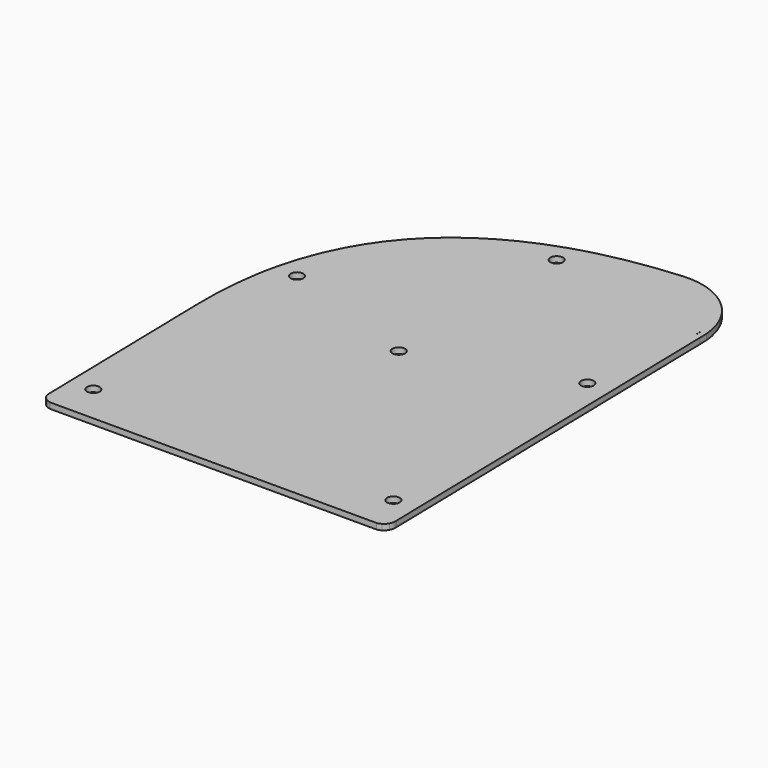
from build123d import *

# Parameters (mm, degrees)
F0_R     = 1.65
F1_DEPTH = 1.5


# Not quite as in the source:
# - the dataset's text gives a spline's control points without its knots; the knots are read off the source's solid
# - a feature names something its author has since deleted; it is built from what else it names


with BuildPart() as f1:
    # F0 (on Top) → F1 (new body)
    with BuildSketch(Plane.XY):
        with BuildLine():
            add(Edge.make_bspline(
                [(-1.4834199291, 56.9861769818), (-24.0434344456, 49.5840490447), (-39.5518296707, 34.0581899342), (-43.7697110627, 8.0514126658)],
                knots=[23.6646194308, 23.6646194308, 23.6646194308, 23.6646194308, 87.6009906021, 87.6009906021, 87.6009906021, 87.6009906021], degree=3))
            Line((-43.7697110627, 8.0514126658), (-43.3999866886, -9.4545040952))
            add(Edge.make_bspline(
                [(-41.6084588868, 11.4552943961), (-41.9131684463, 10.0195533179), (-43.0811996644, 3.5961523714), (-43.5251604122, -3.527708515), (-43.3999866886, -9.4545040952)],
                knots=[0.8378421155, 0.8378421155, 0.8378421155, 0.8378421155, 0.875, 1, 1, 1, 1], degree=3))
            ThreePointArc((-41.6084588868, 11.4552943961), (-41.6746745213, 14.1216598486), (-40.360654899, 16.442703077))
            add(Edge.make_bspline(
                [(-3.9361636907, 54.5413772398), (-7.7396177388, 53.1307994352), (-15.2958477205, 49.6198124705), (-25.1166954602, 42.4854415502), (-33.2620494576, 33.0539884408), (-37.9347962076, 23.9582519777), (-39.9020549062, 18.0232145314), (-40.360654899, 16.442703077)],
                knots=[0.2629122118, 0.2629122118, 0.2629122118, 0.2629122118, 0.375, 0.5, 0.625, 0.75, 0.7934924029, 0.7934924029, 0.7934924029, 0.7934924029], degree=3))
            ThreePointArc((-3.9361636907, 54.5413772398), (-1.5789362683, 56.2022473749), (1.3034460345, 56.2852111481))
            add(Edge.make_bspline(
                [(3.7948607758, 56.9861769817), (2.9552380235, 56.7627416597), (2.1246988708, 56.5291170771), (1.3034460345, 56.2852111481)],
                knots=[0.1898045831, 0.1898045831, 0.1898045831, 0.1898045831, 0.2127848006, 0.2127848006, 0.2127848006, 0.2127848006], degree=3))
            Line((3.7948607758, 56.9861769818), (-1.4834199291, 56.9861769818))
        make_face()
        with BuildLine():
            add(Edge.make_bspline(
                [(-40.360654899, 16.442703077), (-40.8282946823, 14.8310370372), (-41.2447734518, 13.1689200516), (-41.6084588868, 11.4552943961)],
                knots=[0.7934924029, 0.7934924029, 0.7934924029, 0.7934924029, 0.8378421155, 0.8378421155, 0.8378421155, 0.8378421155], degree=3))
            ThreePointArc((-41.6084588868, 11.4552943961), (-36.6028372853, 7.9130121651), (-31.9301505005, 11.884159258))
            ThreePointArc((-31.9301505005, 11.884159258), (-31.8507431164, 12.393400412), (-31.8241799079, 12.9081105068))
            ThreePointArc((-31.8241799079, 12.9081105068), (-34.9113776383, 17.5277628181), (-40.360654899, 16.442703077))
        make_face()
        with Locations((-36.8241799079, 12.9081105068)):
            Circle(F0_R, mode=Mode.SUBTRACT)
        with BuildLine():
            ThreePointArc((-40.360654899, 16.442703077), (-41.6746745213, 14.1216598486), (-41.6084588868, 11.4552943961))
            add(Edge.make_bspline(
                [(-40.360654899, 16.442703077), (-40.8282946823, 14.8310370372), (-41.2447734518, 13.1689200516), (-41.6084588868, 11.4552943961)],
                knots=[0.7934924029, 0.7934924029, 0.7934924029, 0.7934924029, 0.8378421155, 0.8378421155, 0.8378421155, 0.8378421155], degree=3))
        make_face()
        with BuildLine():
            ThreePointArc((-4.0125837516, 2.9831479408), (-4.2957315609, 2.5586501044), (-4.534139997, 2.1075043268))
            ThreePointArc((-4.534139997, 2.1075043268), (-1.0791895142, -4.8821460438), (5, 0))
            ThreePointArc((5, 0), (4.9178269212, 0.9027615264), (4.6740086506, 1.7758499751))
            ThreePointArc((4.6740086506, 1.7758499751), (4.4710674532, 2.2382037059), (4.2225292185, 2.6777316891))
            ThreePointArc((4.2225292185, 2.6777316891), (0.1853079774, 4.9965649154), (-4.0125837516, 2.9831479408))
        make_face()
        Circle(F0_R, mode=Mode.SUBTRACT)
        with BuildLine():
            ThreePointArc((33.856602495, 11.8901119011), (38.3087519579, 7.9829804344), (43.3659270117, 11.0671807542))
            Line((43.3659270117, 11.0671807542), (43.281700799, 15.0551706498))
            ThreePointArc((43.281700799, 15.0551706498), (37.6421734995, 17.842387831), (33.7401541423, 12.9081105068))
            ThreePointArc((33.7401541423, 12.9081105068), (33.7722325318, 12.3961204004), (33.856602495, 11.8901119011))
        make_face()
        with Locations((38.8260431298, 12.9081105068)):
            Circle(F0_R, mode=Mode.SUBTRACT)
        with BuildLine():
            Line((43.281700799, 15.0551706498), (43.3659270117, 11.0671807542))
            ThreePointArc((43.3659270117, 11.0671807542), (43.6454694966, 11.9975237522), (43.7398377061, 12.9643622786))
            ThreePointArc((43.7398377061, 12.9643622786), (43.623960732, 14.0345689258), (43.281700799, 15.0551706498))
        make_face()
        with BuildLine():
            Line((43.3659270117, 11.0671807542), (44.6495853815, -49.7121947628))
            ThreePointArc((44.6495853815, -49.7121947628), (45.057929388, -50.8167509251), (45.1966083023, -51.9861769818))
            ThreePointArc((45.1966083023, -51.9861769818), (45.0815382797, -53.0526942652), (44.7416246559, -54.0701218815))
            Line((44.7416246559, -54.0701218815), (44.7906830466, -56.3929660398))
            ThreePointArc((44.7906830466, -56.3929660398), (45.8531698465, -57.3651583436), (46.3401743003, -58.7204674365))
            Line((46.3401743003, -58.7204674365), (44.1920061045, 42.9922035609))
            ThreePointArc((44.1920061045, 42.9922035609), (43.7876646895, 39.7863466035), (42.8245210763, 36.7019722436))
            Line((42.8245210763, 36.7019722436), (43.281700799, 15.0551706498))
            ThreePointArc((43.281700799, 15.0551706498), (43.623960732, 14.0345689258), (43.7398377061, 12.9643622786))
            ThreePointArc((43.7398377061, 12.9643622786), (43.6454694966, 11.9975237522), (43.3659270117, 11.0671807542))
        make_face()
        with BuildLine():
            ThreePointArc((42.8245210763, 36.7019722436), (43.7876646895, 39.7863466035), (44.1920061045, 42.9922035609))
            Line((44.1920061045, 42.9922035609), (44.1473284715, 45.1076251571))
            ThreePointArc((44.1473284715, 45.1076251571), (43.6079928038, 48.2935516862), (42.5154823554, 51.3345107013))
            Line((42.5154823554, 51.3345107013), (42.6486009917, 45.0315349493))
            ThreePointArc((42.6486009917, 45.0315349493), (42.6904501625, 44.3488552909), (42.704407636, 43.6650365591))
            ThreePointArc((42.704407636, 43.6650365591), (42.7011560215, 43.3349282258), (42.6914024401, 43.0049479956))
            Line((42.6914024401, 43.0049479956), (42.8245210763, 36.7019722436))
        make_face()
        with BuildLine():
            ThreePointArc((42.5154823554, 51.3345107013), (40.7462901657, 54.3570465919), (38.43254048, 56.9861769818))
            Line((38.43254048, 56.9861769818), (36.1139913688, 56.9861769818))
            ThreePointArc((36.1139913688, 56.9861769818), (40.6509720914, 51.7028823031), (42.6486009917, 45.0315349493))
            Line((42.6486009917, 45.0315349493), (42.5154823554, 51.3345107013))
        make_face()
        with BuildLine():
            add(Edge.make_bspline(
                [(24.7414019258, 61.8833889583), (24.6406996854, 61.8759974959), (24.5400748401, 61.8685045119), (24.4395276097, 61.8609098839)],
                knots=[1.1865276968, 1.1865276968, 1.1865276968, 1.1865276968, 1.425041868, 1.425041868, 1.425041868, 1.425041868], degree=3))
            ThreePointArc((24.4395276097, 61.8609098839), (20.5940502811, 61.1210933261), (16.9947819167, 59.5782739378))
            add(Edge.make_bspline(
                [(24.5558527888, 60.365406788), (21.9807579148, 60.170918351), (19.4591236125, 59.9091209792), (16.9947819167, 59.5782739378)],
                knots=[0.0141040109, 0.0141040109, 0.0141040109, 0.0141040109, 0.0753203459, 0.0753203459, 0.0753203459, 0.0753203459], degree=3))
            ThreePointArc((24.5558527888, 60.365406788), (24.7014970491, 60.3768935027), (24.8472359143, 60.3871100752))
            ThreePointArc((24.8472359143, 60.3871100752), (30.7889811323, 59.7082164359), (36.1139913688, 56.9861769818))
            Line((36.1139913688, 56.9861769818), (38.43254048, 56.9861769818))
            ThreePointArc((38.43254048, 56.9861769818), (32.0955113167, 60.8565088809), (24.7414019258, 61.8833889583))
        make_face()
        with BuildLine():
            add(Edge.make_bspline(
                [(24.4395276097, 61.8609098839), (15.0642862312, 61.1527703288), (6.3638379536, 59.5609273996), (-1.4834199291, 56.9861769818)],
                knots=[1.425041868, 1.425041868, 1.425041868, 1.425041868, 23.6646194308, 23.6646194308, 23.6646194308, 23.6646194308], degree=3))
            Line((-1.4834199291, 56.9861769818), (3.7948607758, 56.9861769818))
            add(Edge.make_bspline(
                [(16.9947819167, 59.5782739378), (12.3860728261, 58.9595375953), (7.9777441733, 58.0993005798), (3.7948607758, 56.9861769817)],
                knots=[0.0753203459, 0.0753203459, 0.0753203459, 0.0753203459, 0.1898045831, 0.1898045831, 0.1898045831, 0.1898045831], degree=3))
            ThreePointArc((16.9947819167, 59.5782739378), (20.5940502811, 61.1210933261), (24.4395276097, 61.8609098839))
        make_face()
        with BuildLine():
            ThreePointArc((5, 51.4580972655), (3.969712217, 54.4980618893), (1.3034460345, 56.2852111481))
            add(Edge.make_bspline(
                [(1.3034460345, 56.2852111481), (-0.0265278019, 55.8902188998), (-1.7851459927, 55.3218605731), (-3.4980160121, 54.7038720098), (-3.9361636907, 54.5413772398)],
                knots=[0.2127848006, 0.2127848006, 0.2127848006, 0.2127848006, 0.25, 0.2629122118, 0.2629122118, 0.2629122118, 0.2629122118], degree=3))
            ThreePointArc((-3.9361636907, 54.5413772398), (-1.6308251817, 46.731533056), (5, 51.4580972655))
        make_face()
        with Locations((0, 51.4580972655)):
            Circle(F0_R, mode=Mode.SUBTRACT)
        with BuildLine():
            add(Edge.make_bspline(
                [(1.3034460345, 56.2852111481), (-0.0265278019, 55.8902188998), (-1.7851459927, 55.3218605731), (-3.4980160121, 54.7038720098), (-3.9361636907, 54.5413772398)],
                knots=[0.2127848006, 0.2127848006, 0.2127848006, 0.2127848006, 0.25, 0.2629122118, 0.2629122118, 0.2629122118, 0.2629122118], degree=3))
            ThreePointArc((1.3034460345, 56.2852111481), (-1.5789362683, 56.2022473749), (-3.9361636907, 54.5413772398))
        make_face()
        with BuildLine():
            Line((-44.8996522607, -9.4861769818), (-43.857959234, -58.8088418975))
            ThreePointArc((-43.857959234, -58.8088418975), (-43.423907092, -57.4454091965), (-42.4076946201, -56.4381047717))
            Line((-42.4076946201, -56.4381047717), (-42.4536350786, -54.2628902097))
            ThreePointArc((-42.4536350786, -54.2628902097), (-43.0009389284, -52.0917532702), (-42.5457909037, -49.8994445807))
            Line((-42.5457909037, -49.8994445807), (-43.3999866886, -9.4545040952))
            Line((-43.3999866886, -9.4545040952), (-43.7697110627, 8.0514126658))
            add(Edge.make_bspline(
                [(-43.7697110627, 8.0514126658), (-44.6436982543, 2.6625484195), (-45.0329161364, -3.1763243502), (-44.8996522607, -9.4861769818)],
                knots=[87.6009906021, 87.6009906021, 87.6009906021, 87.6009906021, 100.8492458966, 100.8492458966, 100.8492458966, 100.8492458966], degree=3))
        make_face()
        with BuildLine():
            ThreePointArc((-42.4536350786, -54.2628902097), (-41.8118478695, -55.2243042636), (-40.9664335917, -56.0126458797))
            ThreePointArc((-40.9664335917, -56.0126458797), (-39.732615879, -56.2327544404), (-38.6963915431, -56.9377317823))
            ThreePointArc((-38.6963915431, -56.9377317823), (-34.7211764635, -55.75921881), (-33.0020536879, -51.9861769818))
            ThreePointArc((-33.0020536879, -51.9861769818), (-36.9340382571, -47.1015743327), (-42.5457909037, -49.8994445807))
            Line((-42.5457909037, -49.8994445807), (-42.4536350786, -54.2628902097))
        make_face()
        with Locations((-38.0020536879, -51.9861769818)):
            Circle(F0_R, mode=Mode.SUBTRACT)
        with BuildLine():
            Line((-43.857959234, -58.8088418975), (-43.8467581028, -59.339199334))
            ThreePointArc((-43.8467581028, -59.339199334), (-43.7200551284, -59.9314469487), (-43.4769800964, -60.4861769818))
            Line((-43.4769800964, -60.4861769818), (-42.3221994709, -60.4861769818))
            Line((-42.3221994709, -60.4861769818), (-42.4076946201, -56.4381047717))
            ThreePointArc((-42.4076946201, -56.4381047717), (-43.423907092, -57.4454091965), (-43.857959234, -58.8088418975))
        make_face()
        with BuildLine():
            ThreePointArc((-43.4769800964, -60.4861769818), (-42.96891188, -61.1492867627), (-42.2976915724, -61.6465906868))
            Line((-42.2976915724, -61.6465906868), (-42.3221994709, -60.4861769818))
            Line((-42.3221994709, -60.4861769818), (-43.4769800964, -60.4861769818))
        make_face()
        with BuildLine():
            ThreePointArc((-42.2976915724, -61.6465906868), (-41.7892239121, -61.8649359932), (-41.2493029391, -61.9861769818))
            Line((-41.2493029391, -61.9861769818), (-40.4802432502, -61.9861769818))
            ThreePointArc((-40.4802432502, -61.9861769818), (-39.1891812794, -61.49937465), (-38.2525660929, -60.4861769818))
            Line((-38.2525660929, -60.4861769818), (-42.3221994709, -60.4861769818))
            Line((-42.3221994709, -60.4861769818), (-42.2976915724, -61.6465906868))
        make_face()
        with BuildLine():
            ThreePointArc((-38.2525660929, -60.4861769818), (-39.1891812794, -61.49937465), (-40.4802432502, -61.9861769818))
            Line((-40.4802432502, -61.9861769818), (42.8588795725, -61.9861769818))
            ThreePointArc((42.8588795725, -61.9861769818), (41.6256295111, -61.4783601673), (40.7343629083, -60.4861769818))
            Line((40.7343629083, -60.4861769818), (-38.2525660929, -60.4861769818))
        make_face()
        with BuildLine():
            ThreePointArc((40.7343629083, -60.4861769818), (41.6256295111, -61.4783601673), (42.8588795725, -61.9861769818))
            Line((42.8588795725, -61.9861769818), (43.8530039724, -61.9861769818))
            ThreePointArc((43.8530039724, -61.9861769818), (44.3949796267, -61.8419625935), (44.9006425936, -61.5993922664))
            Line((44.9006425936, -61.5993922664), (44.8771315242, -60.4861769818))
            Line((44.8771315242, -60.4861769818), (40.7343629083, -60.4861769818))
        make_face()
        with BuildLine():
            Line((44.7906830466, -56.3929660398), (44.8771315242, -60.4861769818))
            Line((44.8771315242, -60.4861769818), (45.9775206366, -60.4861769818))
            ThreePointArc((45.9775206366, -60.4861769817), (46.2357482904, -59.8683050946), (46.3504824841, -59.2085450967))
            Line((46.3504824841, -59.2085450967), (46.3401743003, -58.7204674365))
            ThreePointArc((46.3401743003, -58.7204674365), (45.8531698465, -57.3651583436), (44.7906830466, -56.3929660398))
        make_face()
        with BuildLine():
            Line((44.8771315242, -60.4861769818), (44.9006425936, -61.5993922664))
            ThreePointArc((44.9006425936, -61.5993922664), (45.5121615367, -61.1134790926), (45.9775206366, -60.4861769817))
            Line((45.9775206366, -60.4861769818), (44.8771315242, -60.4861769818))
        make_face()
        with BuildLine():
            ThreePointArc((44.6495853815, -49.7121947628), (35.6747286545, -49.8524936757), (41.2725763461, -56.8690340111))
            ThreePointArc((41.2725763461, -56.8690340111), (42.1278630999, -56.2905225817), (43.1286349994, -56.0362658014))
            ThreePointArc((43.1286349994, -56.0362658014), (44.062222571, -55.1574584776), (44.7416246559, -54.0701218815))
            Line((44.7416246559, -54.0701218815), (44.6495853815, -49.7121947628))
        make_face()
        with Locations((40.1966083023, -51.9861769818)):
            Circle(F0_R, mode=Mode.SUBTRACT)
        with BuildLine():
            ThreePointArc((41.2725763461, -56.8690340111), (40.3886103094, -58.5861173938), (40.7343629083, -60.4861769818))
            Line((40.7343629083, -60.4861769818), (44.8771315242, -60.4861769818))
            Line((44.8771315242, -60.4861769818), (44.7906830466, -56.3929660398))
            ThreePointArc((44.7906830466, -56.3929660398), (43.9854521247, -56.0944327255), (43.1286349994, -56.0362658014))
            ThreePointArc((43.1286349994, -56.0362658014), (42.2434060899, -56.5480426984), (41.2725763461, -56.8690340111))
        make_face()
        with BuildLine():
            ThreePointArc((44.7416246559, -54.0701218815), (44.062222571, -55.1574584776), (43.1286349994, -56.0362658014))
            ThreePointArc((43.1286349994, -56.0362658014), (43.9854521247, -56.0944327255), (44.7906830466, -56.3929660398))
            Line((44.7906830466, -56.3929660398), (44.7416246559, -54.0701218815))
        make_face()
        with BuildLine():
            ThreePointArc((43.1286349994, -56.0362658014), (42.1278630999, -56.2905225817), (41.2725763461, -56.8690340111))
            ThreePointArc((41.2725763461, -56.8690340111), (42.2434060899, -56.5480426984), (43.1286349994, -56.0362658014))
        make_face()
        with BuildLine():
            ThreePointArc((45.1966083023, -51.9861769818), (45.057929388, -50.8167509251), (44.6495853815, -49.7121947628))
            Line((44.6495853815, -49.7121947628), (44.7416246559, -54.0701218815))
            ThreePointArc((44.7416246559, -54.0701218815), (45.0815382797, -53.0526942652), (45.1966083023, -51.9861769818))
        make_face()
        with BuildLine():
            ThreePointArc((-42.5457909037, -49.8994445807), (-43.0009389284, -52.0917532702), (-42.4536350786, -54.2628902097))
            Line((-42.4536350786, -54.2628902097), (-42.5457909037, -49.8994445807))
        make_face()
        with BuildLine():
            ThreePointArc((-38.6963915431, -56.9377317823), (-39.732615879, -56.2327544404), (-40.9664335917, -56.0126458797))
            ThreePointArc((-40.9664335917, -56.0126458797), (-39.8889823808, -56.6164577625), (-38.6963915431, -56.9377317823))
        make_face()
        with BuildLine():
            Line((-42.3221994709, -60.4861769818), (-38.2525660929, -60.4861769818))
            ThreePointArc((-38.2525660929, -60.4861769818), (-37.9633406032, -59.7736086221), (-37.8647730947, -59.0109229088))
            ThreePointArc((-37.8647730947, -59.0109229088), (-38.0804289479, -57.8940398922), (-38.6963915431, -56.9377317823))
            ThreePointArc((-38.6963915431, -56.9377317823), (-39.8889823808, -56.6164577625), (-40.9664335917, -56.0126458797))
            ThreePointArc((-40.9664335917, -56.0126458797), (-41.7141353992, -56.1336701087), (-42.4076946201, -56.4381047717))
            Line((-42.4076946201, -56.4381047717), (-42.3221994709, -60.4861769818))
        make_face()
        with BuildLine():
            Line((-42.4536350786, -54.2628902097), (-42.4076946201, -56.4381047717))
            ThreePointArc((-42.4076946201, -56.4381047717), (-41.7141353992, -56.1336701087), (-40.9664335917, -56.0126458797))
            ThreePointArc((-40.9664335917, -56.0126458797), (-41.8118478695, -55.2243042636), (-42.4536350786, -54.2628902097))
        make_face()
        with BuildLine():
            Line((4.6740086506, 1.7758499751), (33.856602495, 11.8901119011))
            ThreePointArc((33.856602495, 11.8901119011), (33.7722325318, 12.3961204004), (33.7401541423, 12.9081105068))
            Line((33.7401541423, 12.9081105068), (4.2225292185, 2.6777316891))
            ThreePointArc((4.2225292185, 2.6777316891), (4.4710674532, 2.2382037059), (4.6740086506, 1.7758499751))
        make_face()
        with BuildLine():
            ThreePointArc((-31.8241799079, 12.9081105068), (-31.8507431164, 12.393400412), (-31.9301505005, 11.884159258))
            Line((-31.9301505005, 11.884159258), (-4.534139997, 2.1075043268))
            ThreePointArc((-4.534139997, 2.1075043268), (-4.2957315609, 2.5586501044), (-4.0125837516, 2.9831479408))
            Line((-4.0125837516, 2.9831479408), (-31.8241799079, 12.9081105068))
        make_face()
        with BuildLine():
            Line((13.4599747919, 56.9861769818), (3.7948607758, 56.9861769818))
            add(Edge.make_bspline(
                [(3.7948607758, 56.9861769817), (2.9552380235, 56.7627416597), (2.1246988708, 56.5291170771), (1.3034460345, 56.2852111481)],
                knots=[0.1898045831, 0.1898045831, 0.1898045831, 0.1898045831, 0.2127848006, 0.2127848006, 0.2127848006, 0.2127848006], degree=3))
            ThreePointArc((1.3034460345, 56.2852111481), (3.969712217, 54.4980618893), (5, 51.4580972655))
            ThreePointArc((5, 51.4580972655), (-1.6308251817, 46.731533056), (-3.9361636907, 54.5413772398))
            add(Edge.make_bspline(
                [(-3.9361636907, 54.5413772398), (-7.7396177388, 53.1307994352), (-15.2958477205, 49.6198124705), (-25.1166954602, 42.4854415502), (-33.2620494576, 33.0539884408), (-37.9347962076, 23.9582519777), (-39.9020549062, 18.0232145314), (-40.360654899, 16.442703077)],
                knots=[0.2629122118, 0.2629122118, 0.2629122118, 0.2629122118, 0.375, 0.5, 0.625, 0.75, 0.7934924029, 0.7934924029, 0.7934924029, 0.7934924029], degree=3))
            ThreePointArc((-40.360654899, 16.442703077), (-34.9113776383, 17.5277628181), (-31.8241799079, 12.9081105068))
            Line((-31.8241799079, 12.9081105068), (-4.0125837516, 2.9831479408))
            ThreePointArc((-4.0125837516, 2.9831479408), (0.1853079774, 4.9965649154), (4.2225292185, 2.6777316891))
            Line((4.2225292185, 2.6777316891), (33.7401541423, 12.9081105068))
            ThreePointArc((33.7401541423, 12.9081105068), (37.6421734995, 17.842387831), (43.281700799, 15.0551706498))
            Line((43.281700799, 15.0551706498), (42.8245210763, 36.7019722436))
            ThreePointArc((42.8245210763, 36.7019722436), (15.5691379077, 28.6425391779), (13.4599747919, 56.9861769817))
        make_face()
        with BuildLine():
            Line((36.1139913688, 56.9861769818), (15.7785239031, 56.9861769818))
            ThreePointArc((15.7785239031, 56.9861769818), (18.2206977798, 28.7938793637), (42.6914024401, 43.0049479956))
            Line((42.6914024401, 43.0049479956), (42.6486009917, 45.0315349493))
            ThreePointArc((42.6486009917, 45.0315349493), (40.6509720914, 51.7028823031), (36.1139913688, 56.9861769818))
        make_face()
        with BuildLine():
            add(Edge.make_bspline(
                [(24.8472359143, 60.3871100752), (24.7500324053, 60.3799711919), (24.6529046285, 60.3727367939), (24.5558527888, 60.365406788)],
                knots=[0.0117968501, 0.0117968501, 0.0117968501, 0.0117968501, 0.0141040109, 0.0141040109, 0.0141040109, 0.0141040109], degree=3))
            ThreePointArc((24.5558527888, 60.365406788), (19.9252576875, 59.3041909814), (15.7785239031, 56.9861769818))
            Line((15.7785239031, 56.9861769818), (36.1139913688, 56.9861769818))
            ThreePointArc((36.1139913688, 56.9861769818), (30.7889811323, 59.7082164359), (24.8472359143, 60.3871100752))
        make_face()
        with BuildLine():
            add(Edge.make_bspline(
                [(16.9947819167, 59.5782739378), (12.3860728261, 58.9595375953), (7.9777441733, 58.0993005798), (3.7948607758, 56.9861769817)],
                knots=[0.0753203459, 0.0753203459, 0.0753203459, 0.0753203459, 0.1898045831, 0.1898045831, 0.1898045831, 0.1898045831], degree=3))
            Line((3.7948607758, 56.9861769818), (13.4599747919, 56.9861769818))
            ThreePointArc((13.4599747919, 56.9861769817), (15.1493083116, 58.3886885079), (16.9947819167, 59.5782739378))
        make_face()
        with BuildLine():
            add(Edge.make_bspline(
                [(24.5558527888, 60.365406788), (21.9807579148, 60.170918351), (19.4591236125, 59.9091209792), (16.9947819167, 59.5782739378)],
                knots=[0.0141040109, 0.0141040109, 0.0141040109, 0.0141040109, 0.0753203459, 0.0753203459, 0.0753203459, 0.0753203459], degree=3))
            ThreePointArc((16.9947819167, 59.5782739378), (15.1493083116, 58.3886885079), (13.4599747919, 56.9861769817))
            Line((13.4599747919, 56.9861769818), (15.7785239031, 56.9861769818))
            ThreePointArc((15.7785239031, 56.9861769818), (19.9252576875, 59.3041909814), (24.5558527888, 60.365406788))
        make_face()
        with BuildLine():
            Line((15.7785239031, 56.9861769818), (13.4599747919, 56.9861769818))
            ThreePointArc((13.4599747919, 56.9861769817), (15.5691379077, 28.6425391779), (42.8245210763, 36.7019722436))
            Line((42.8245210763, 36.7019722436), (42.6914024401, 43.0049479956))
            ThreePointArc((42.6914024401, 43.0049479956), (18.2206977798, 28.7938793637), (15.7785239031, 56.9861769818))
        make_face()
        with BuildLine():
            ThreePointArc((-37.8647730947, -59.0109229088), (-37.9633406032, -59.7736086221), (-38.2525660929, -60.4861769818))
            Line((-38.2525660929, -60.4861769818), (40.7343629083, -60.4861769818))
            ThreePointArc((40.7343629083, -60.4861769818), (40.3886103094, -58.5861173938), (41.2725763461, -56.8690340111))
            ThreePointArc((41.2725763461, -56.8690340111), (35.6747286545, -49.8524936757), (44.6495853815, -49.7121947628))
            Line((44.6495853815, -49.7121947628), (43.3659270117, 11.0671807542))
            ThreePointArc((43.3659270117, 11.0671807542), (38.3087519579, 7.9829804344), (33.856602495, 11.8901119011))
            Line((33.856602495, 11.8901119011), (4.6740086506, 1.7758499751))
            ThreePointArc((4.6740086506, 1.7758499751), (4.9178269212, 0.9027615264), (5, 0))
            ThreePointArc((5, 0), (-1.0791895142, -4.8821460438), (-4.534139997, 2.1075043268))
            Line((-4.534139997, 2.1075043268), (-31.9301505005, 11.884159258))
            ThreePointArc((-31.9301505005, 11.884159258), (-36.6028372853, 7.9130121651), (-41.6084588868, 11.4552943961))
            add(Edge.make_bspline(
                [(-41.6084588868, 11.4552943961), (-41.9131684463, 10.0195533179), (-43.0811996644, 3.5961523714), (-43.5251604122, -3.527708515), (-43.3999866886, -9.4545040952)],
                knots=[0.8378421155, 0.8378421155, 0.8378421155, 0.8378421155, 0.875, 1, 1, 1, 1], degree=3))
            Line((-43.3999866886, -9.4545040952), (-42.5457909037, -49.8994445807))
            ThreePointArc((-42.5457909037, -49.8994445807), (-36.9340382571, -47.1015743327), (-33.0020536879, -51.9861769818))
            ThreePointArc((-33.0020536879, -51.9861769818), (-34.7211764635, -55.75921881), (-38.6963915431, -56.9377317823))
            ThreePointArc((-38.6963915431, -56.9377317823), (-38.0804289479, -57.8940398922), (-37.8647730947, -59.0109229088))
        make_face()
    extrude(amount=F1_DEPTH)


solid = f1.part
